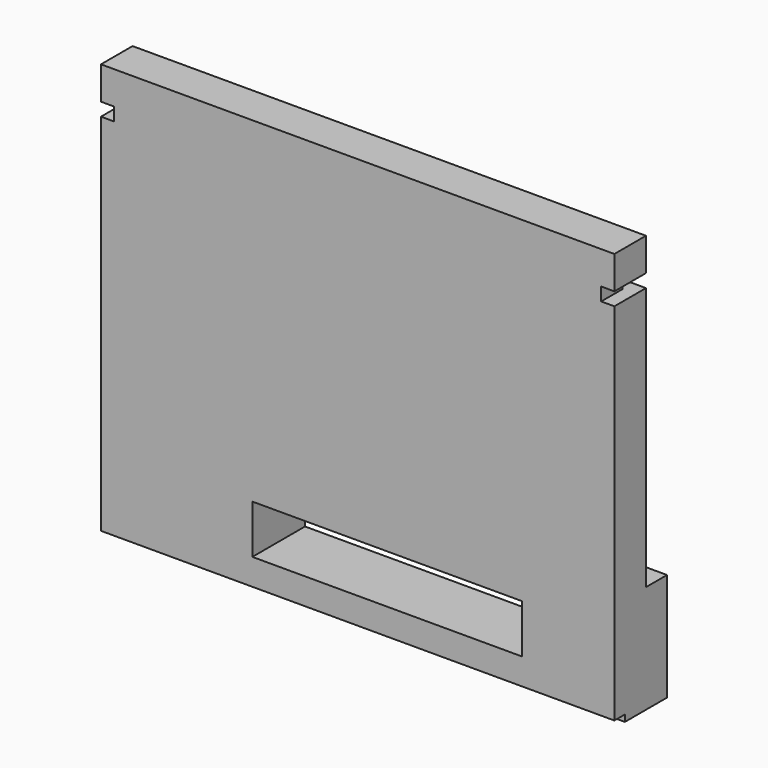
from build123d import *

# Parameters (mm, degrees)
F0_W      = 3900
F0_H      = 400
F1_DEPTH  = 50
F2_W      = 3900
F2_H      = 500
F3_DEPTH  = 200
F4_W      = 700
F4_H      = 500
F4_W_2    = 1150
F5_DEPTH  = 370
F6_W      = 3900
F6_H      = 500
F7_DEPTH  = 200
F8_W      = 3900
F8_H      = 300
F9_DEPTH  = 2000
F10_W     = 3700
F10_H     = 200
F11_DEPTH = 100
F12_W     = 3900
F12_H     = 300
F13_DEPTH = 250


# Not quite as in the source:
# - a feature names something its author has since deleted; it is built from what else it names


with BuildPart() as f1:
    # F0 (on Top) → F1 (new body)
    with BuildSketch(Plane.XY):
        with Locations((0, -181.2429684355)):
            Rectangle(F0_W, F0_H)
    extrude(amount=F1_DEPTH)

    # F2 (on face) → F3 (join)
    with BuildSketch(Plane.XY.offset(50)):
        with Locations((0, -231.2429684355)):
            Rectangle(F2_W, F2_H)
    extrude(amount=F3_DEPTH)

    # F4 (on face) → F5 (join)
    with BuildSketch(Plane.XY.offset(250)):
        with Locations((1600, -231.2429684355)):
            Rectangle(F4_W, F4_H)
        with Locations((-1375, -231.2429684355)):
            Rectangle(F4_W_2, F4_H)
    extrude(amount=F5_DEPTH)

    # F6 (on face) → F7 (join)
    with BuildSketch(Plane.XY.offset(620)):
        with Locations((0, -231.2429684355)):
            Rectangle(F6_W, F6_H)
    extrude(amount=F7_DEPTH)

    # F8 (on face) → F9 (join)
    with BuildSketch(Plane.XY.offset(820)):
        with Locations((0, -331.2429684355)):
            Rectangle(F8_W, F8_H)
    extrude(amount=F9_DEPTH)

    # F10 (on face) → F11 (join)
    with BuildSketch(Plane.XY.offset(2820)):
        with Locations((0, -381.2429684355)):
            Rectangle(F10_W, F10_H)
    extrude(amount=F11_DEPTH)

    # F12 (on face) → F13 (join)
    with BuildSketch(Plane.XY.offset(2920)):
        with Locations((0, -331.2429684355)):
            Rectangle(F12_W, F12_H)
    extrude(amount=F13_DEPTH)


solid = f1.part
